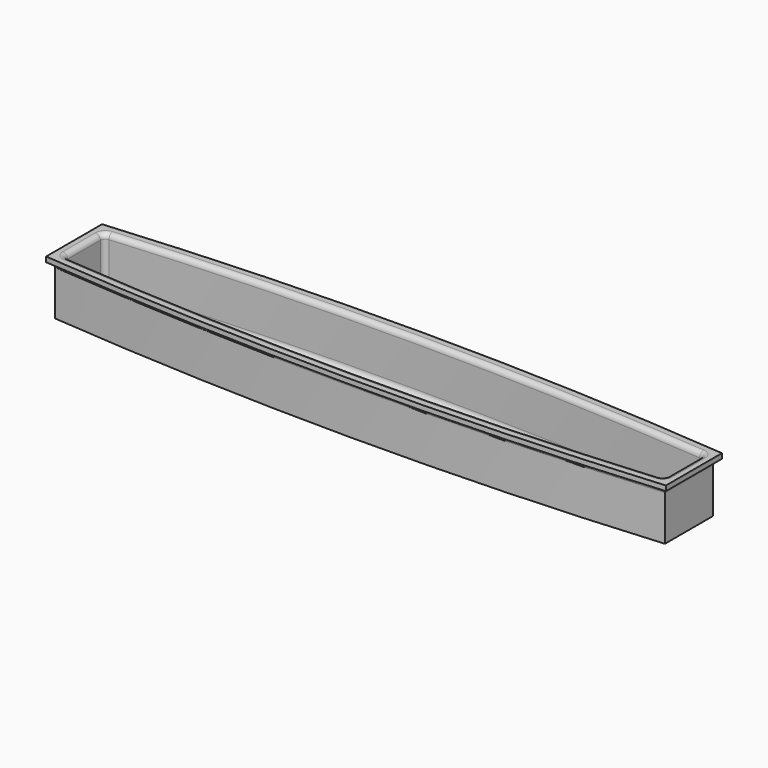
from build123d import *

# Parameters (mm, degrees)
F1_DEPTH = 2.54
F2_DEPTH = 27.94
F4_DEPTH = 2.54
F5_R     = 2.53999


# Not quite as in the source:
# - a fillet or chamfer is up to 0.001 mm smaller than in the source, because OpenCascade refuses the exact size


with BuildPart() as f1:
    # F0 (on Top) → F1 (new body)
    with BuildSketch(Plane.XY):
        with BuildLine():
            Line((0, 25.4), (0, 0))
            ThreePointArc((0, 0), (152.4, -6.35), (304.8, 0))
            Line((304.8, 0), (304.8, 25.4))
            ThreePointArc((304.8, 25.4), (152.4, 31.75), (0, 25.4))
        make_face()
    extrude(amount=F1_DEPTH)

    # F0 (on Top) → F2 (join)
    with BuildSketch(Plane.XY):
        with BuildLine():
            Line((-2.54, 27.94), (-2.54, -2.54))
            ThreePointArc((-2.54, -2.54), (152.4, -9.0943273232), (307.34, -2.54))
            Line((307.34, -2.54), (307.34, 27.94))
            ThreePointArc((307.34, 27.94), (152.4, 34.4943273232), (-2.54, 27.94))
        make_face()
        with BuildLine():
            ThreePointArc((304.8, 0), (152.4, -6.35), (0, 0))
            Line((0, 0), (0, 25.4))
            ThreePointArc((0, 25.4), (152.4, 31.75), (304.8, 25.4))
            Line((304.8, 25.4), (304.8, 0))
        make_face(mode=Mode.SUBTRACT)
    extrude(amount=F2_DEPTH)

    # F3 (on face) → F4 (join)
    with BuildSketch(Plane.XY.offset(27.94)):
        with BuildLine():
            ThreePointArc((309.88, 30.48), (152.4, 37.2416066482), (-5.08, 30.48))
            Line((-5.08, 30.48), (-5.08, -5.08))
            ThreePointArc((-5.08, -5.08), (152.4, -11.8416066482), (309.88, -5.08))
            Line((309.88, -5.08), (309.88, 30.48))
        make_face()
        with BuildLine():
            ThreePointArc((-2.54, 27.94), (152.4, 34.4943273232), (307.34, 27.94))
            Line((307.34, 27.94), (307.34, -2.54))
            ThreePointArc((307.34, -2.54), (152.4, -9.0943273232), (-2.54, -2.54))
            Line((-2.54, -2.54), (-2.54, 27.94))
        make_face(mode=Mode.SUBTRACT)
    extrude(amount=-F4_DEPTH)

    # F5 (radius 2.54 in the source; OpenCascade refuses exactly that, so slightly less here)
    f5_edges = [f1.edges().sort_by_distance(p)[0] for p in [
        (152.4, -9.094327, 25.4),
        (307.34, 12.7, 25.4),
        (152.4, 34.494327, 25.4),
        (-2.54, 12.7, 25.4),
        (0, 25.4, 15.24),
        (152.4, 31.75, 2.54),
        (0, 12.7, 2.54),
        (0, 0, 15.24),
        (304.8, 12.7, 2.54),
        (152.4, -6.35, 2.54),
        (304.8, 25.4, 15.24),
        (304.8, 0, 15.24),
        (152.4, 31.75, 27.94),
        (0, 12.7, 27.94),
        (304.8, 12.7, 27.94),
        (152.4, -6.35, 27.94),
    ]]
    fillet(f5_edges, radius=F5_R)


solid = f1.part
